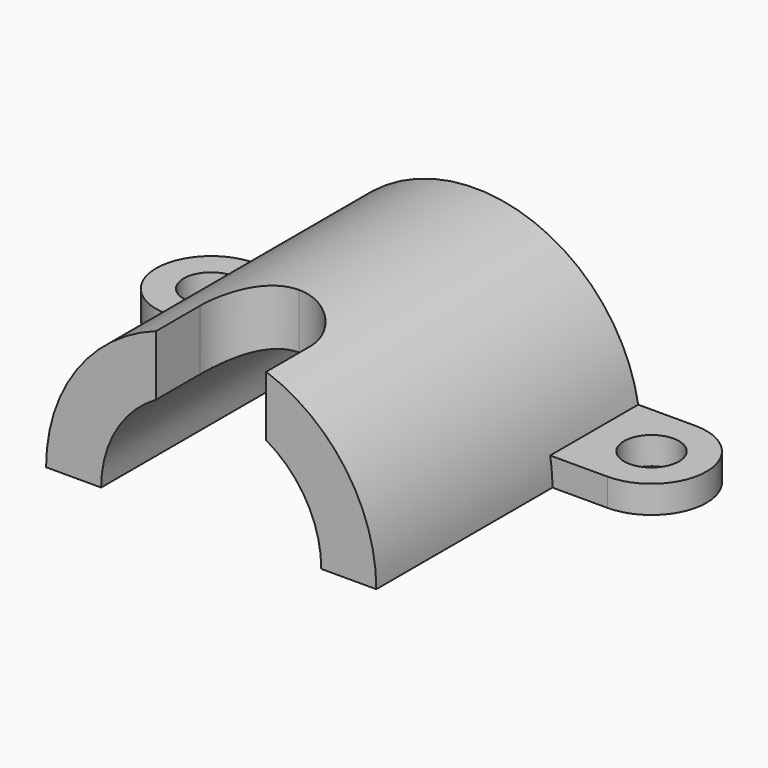
from build123d import *

# Parameters (mm, degrees)
F1_DEPTH  = 60
F3_DEPTH  = 5
F4_R      = 5
F5_DEPTH  = 30.001
F6_W      = 20
F6_H      = 20
F7_DEPTH  = 30.001
F8_R      = 9.999
F10_DEPTH = 60.0010001


# Not quite as in the source:
# - a fillet or chamfer is up to 0.001 mm smaller than in the source, because OpenCascade refuses the exact size


with BuildPart() as f1:
    # F0 (on Front) → F1 (new body)
    with BuildSketch(Plane.XZ):
        with BuildLine():
            Line((-30, 0), (30, 0))
            ThreePointArc((30, 0), (0, 30), (-30, 0))
        make_face()
    extrude(amount=F1_DEPTH)

    # F2 (on Top) → F3 (join)
    with BuildSketch(Plane.XY):
        with BuildLine():
            Line((40, 0), (-40, 0))
            ThreePointArc((-40, 0), (-50, -10), (-40, -20))
            Line((-40, -20), (40, -20))
            ThreePointArc((40, -20), (50, -10), (40, 0))
        make_face()
    extrude(amount=F3_DEPTH)

    # F4 (on Top) → F5 (cut, through all)
    with BuildSketch(Plane.XY):
        with Locations((-40, -10)):
            Circle(F4_R)
        with Locations((40, -10)):
            Circle(F4_R)
    extrude(amount=F5_DEPTH, mode=Mode.SUBTRACT)

    # F6 (on Top) → F7 (cut, through all)
    with BuildSketch(Plane.XY):
        with Locations((0, -50.0372105837)):
            Rectangle(F6_W, F6_H)
    extrude(amount=F7_DEPTH, mode=Mode.SUBTRACT)

    # F8 (radius 10 in the source; OpenCascade refuses exactly that, so slightly less here)
    f8_edges = [f1.edges().sort_by_distance(p)[0] for p in [
        (-10, -40.037211, 14.142136),
        (10, -40.037211, 14.142136),
    ]]
    fillet(f8_edges, radius=F8_R)

    # F9 (on face) → F10 (cut, through all)
    with BuildSketch(Plane(origin=(0, 0, 0), x_dir=(-1, 0, 0), z_dir=(0, 1, 0))):
        with BuildLine():
            Line((-20, 0), (20, 0))
            ThreePointArc((20, 0), (0, 20), (-20, 0))
        make_face()
    extrude(amount=-F10_DEPTH, mode=Mode.SUBTRACT)


solid = f1.part
